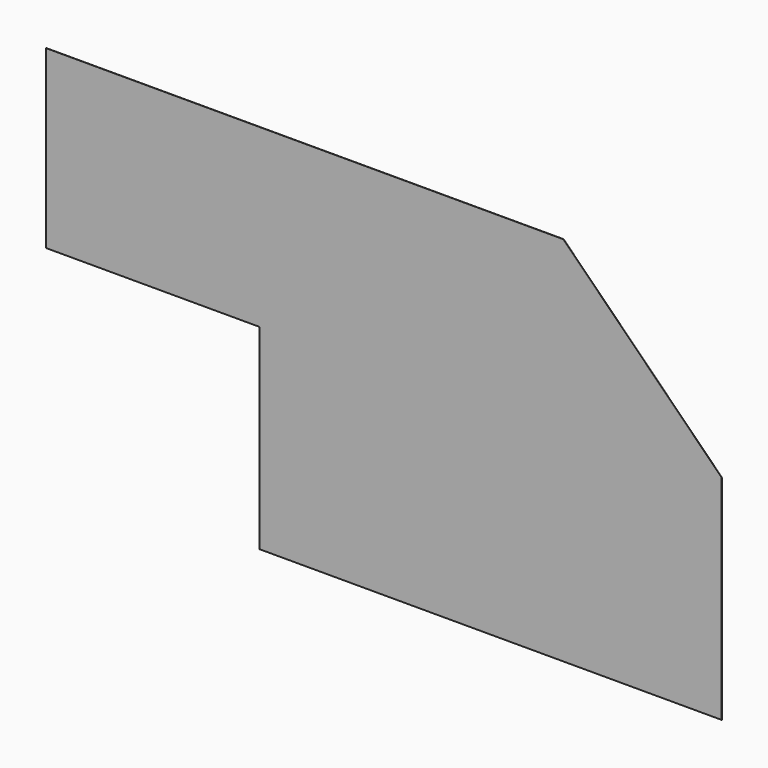
from build123d import *

# Parameters (mm, degrees)
F1_DEPTH = 0.3135802469


# Not quite as in the source:
# - a length typed as a fraction of an inch, garbled in the dataset ("3 / 203.2 mm" for 3/8 in), is restored


with BuildPart() as f1:
    # F0 (on Front) → F1 (new body)
    with BuildSketch(Plane.XZ):
        Polygon((-447.4302810179, 374.6167815521), (-447.4302810179, 123.1567815521), (-142.387826767, 123.1567815521), (-142.387826767, -156.4856726988), (518.012173233, -156.4856726988), (518.012173233, 148.3143273012), (291.7097189821, 374.6167815521), align=None)
    extrude(amount=F1_DEPTH)


solid = f1.part
